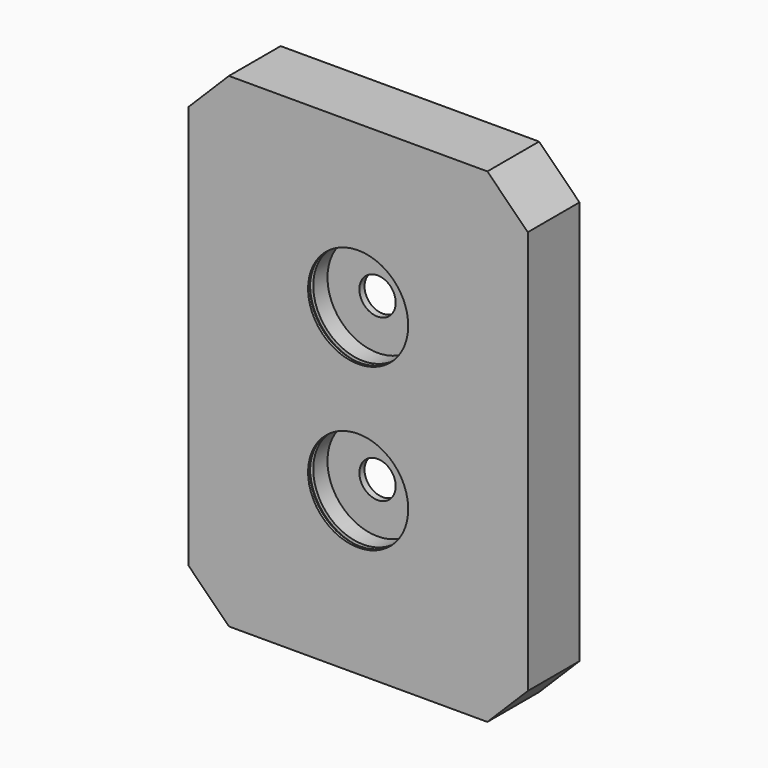
from build123d import *

# Parameters (mm, degrees)
F1_DEPTH = 20
F2_W     = 3.0358287096
F2_H     = 31
F2_W_2   = 4
F2_H_2   = 11.25


# Not quite as in the source:
# - a pattern or mirror of a feature is missing from the dataset's text; its kind, count and spacing are read off the source's solid


with BuildPart() as f1:
    # F0 (on Front) → F1 (new body, symmetric)
    with BuildSketch(Plane.XZ):
        Polygon((80, 150), (-80, 150), (-105, 125), (-105, -125), (-80, -150), (80, -150), (105, -125), (105, 125), align=None)
    extrude(amount=F1_DEPTH, both=True)

    # F2 (on Right) → F3 (revolve, cut)
    with BuildSketch(Plane.YZ):
        with Locations((-20.0179143548, 65.5)):
            Rectangle(F2_W, F2_H)
        Polygon((-18.5, 81), (-18.5, 50), (-16, 50), (-16, 81), (-16, 83), (-18.5, 83), align=None)
        Polygon((-16, 81), (-16, 50), (-5, 50), (-5, 61.25), (-5, 81), align=None)
        with Locations((-3, 55.625)):
            Rectangle(F2_W_2, F2_H_2)
        Polygon((-1, 61.25), (-1, 50), (34.8119065166, 50), (34.8119065166, 86), (-1, 86), align=None)
    f3 = revolve(axis=Axis((0, 5.6746993214, 50), (0, 1, 0)), mode=Mode.SUBTRACT)

    # F3_copies: F3 across plane
    add(f3.mirror(Plane(origin=(0, 0, 0), x_dir=(-1, 0, 0), z_dir=(0, 0, -1))), mode=Mode.SUBTRACT)


solid = f1.part
